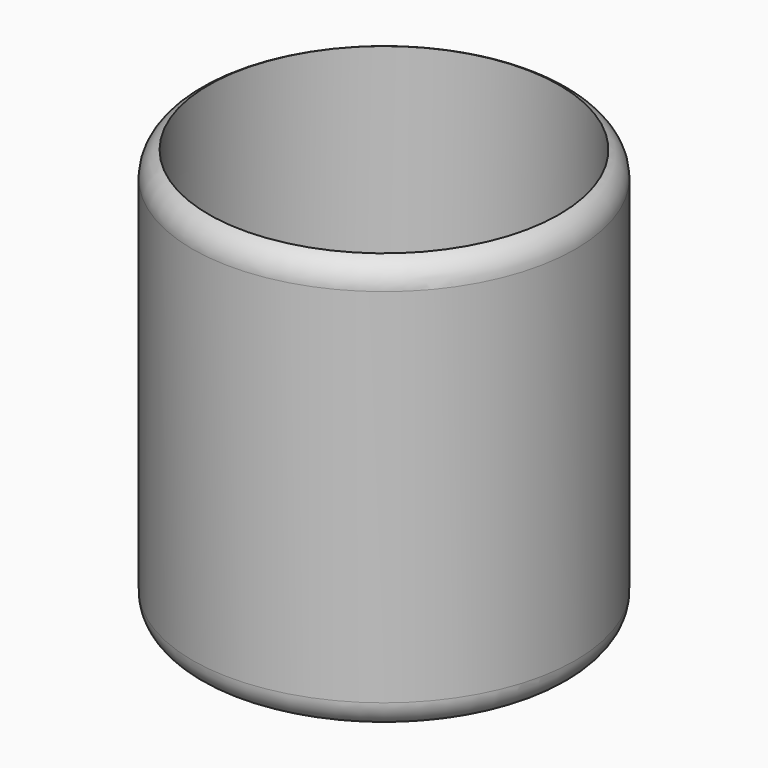
from build123d import *

# Parameters (mm, degrees)
F0_R     = 35.1918039157
F0_R_2   = 32.1953483685
F1_DEPTH = 76.2
F2_R     = 32.3619663376
F3_DEPTH = 25.4
F4_DEPTH = 20.32


# Not quite as in the source:
# - a fillet or chamfer that OpenCascade refuses, or shapes differently, is made with other operations: its cross-section is extruded or revolved along the edge and cut away or added


with BuildPart() as f1:
    # F0 (on Top) → F1 (new body)
    with BuildSketch(Plane.XY):
        Circle(F0_R)
        Circle(F0_R_2, mode=Mode.SUBTRACT)
    extrude(amount=F1_DEPTH)

    # F2 (on Top) → F3 (join)
    with BuildSketch(Plane.XY):
        Circle(F2_R)
    extrude(amount=F3_DEPTH)

    # F4 (cut): a face of the model
    f4_faces = [f1.faces().sort_by_distance(p)[0] for p in [
        (0, 0, 25.4),
    ]]
    extrude(f4_faces, amount=-F4_DEPTH, mode=Mode.SUBTRACT)

    # F5: fillet of radius 5.08 on 2 edges, made by hand

    # F5_s1 → F5_t2 (revolve, cut)
    with BuildSketch(Plane.XZ):
        with BuildLine():
            ThreePointArc((35.1918039157, 71.5669402644), (34.377410896, 74.3257438258), (32.1953483685, 76.2))
            Line((32.1953483685, 76.2), (32.2370192575, 76.2926611947))
            ThreePointArc((32.2370192575, 76.2926611947), (33.6935761421, 76.3016), (35.1918039157, 76.3016))
            Line((35.1918039157, 76.3016), (35.2934039157, 76.2))
            Line((35.2934039157, 76.2), (35.2934039157, 71.5669402644))
            Line((35.2934039157, 71.5669402644), (35.1918039157, 71.5669402644))
        make_face()
    revolve(axis=Axis((0, 0, 76.2), (0, 0, 1)), mode=Mode.SUBTRACT)

    # F5_s3 → F5_t4 (revolve, cut)
    with BuildSketch(Plane.XZ):
        with BuildLine():
            ThreePointArc((35.1918039157, 5.08), (33.7039063642, 1.4878975516), (30.1118039157, 0))
            Line((30.1118039157, 0), (30.1118039157, -0.1016))
            Line((30.1118039157, -0.1016), (35.2934039157, -0.1016))
            Line((35.2934039157, -0.1016), (35.2934039157, 5.08))
            Line((35.2934039157, 5.08), (35.1918039157, 5.08))
        make_face()
    revolve(axis=Axis((0, 0, 0), (0, 0, 1)), mode=Mode.SUBTRACT)


solid = f1.part
